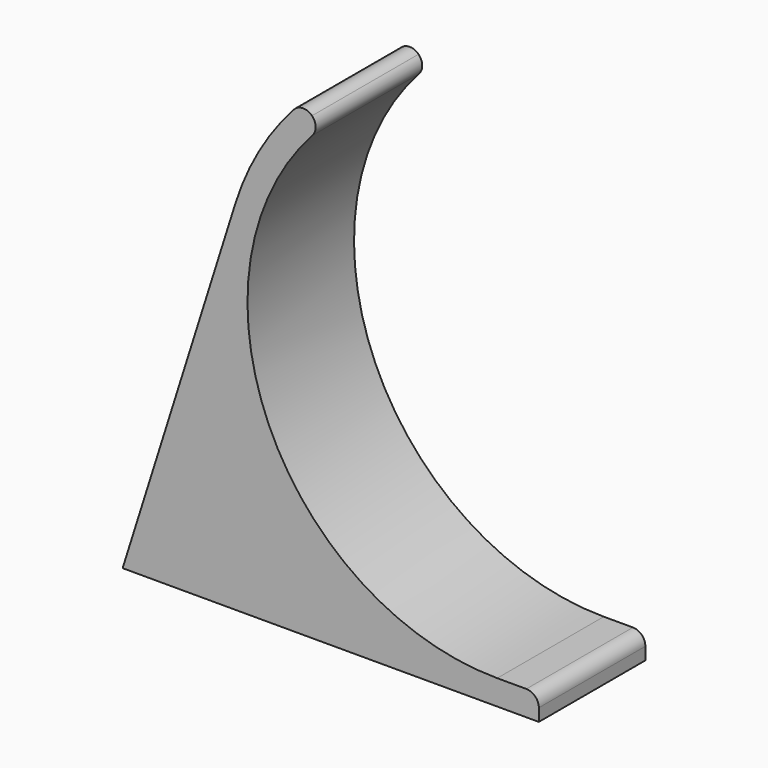
from build123d import *

# Parameters (mm, degrees)
F1_DEPTH = 16
F2_R     = 1.49999


# Not quite as in the source:
# - a fillet or chamfer is up to 0.001 mm smaller than in the source, because OpenCascade refuses the exact size


with BuildPart() as f1:
    # F0 (on Front) → F1 (new body)
    with BuildSketch(Plane.XZ):
        with BuildLine():
            ThreePointArc((0, -33), (-26.6113648632, -19.5150008997), (-31.4739884393, 9.9190751445))
            Line((-31.4739884393, 9.9190751445), (-45, -33))
            Line((-45, -33), (0, -33))
        make_face()
        with BuildLine():
            Line((5, -30), (0, -30))
            ThreePointArc((0, -30), (-27.7163859753, -11.480502971), (-21.2132034356, 21.2132034356))
            Line((-21.2132034356, 21.2132034356), (-23.3345237792, 23.3345237792))
            ThreePointArc((-23.3345237792, 23.3345237792), (-28.213238354, 17.1176278024), (-31.4739884393, 9.9190751445))
            ThreePointArc((-31.4739884393, 9.9190751445), (-26.6113648632, -19.5150008997), (0, -33))
            ThreePointArc((0, -33), (2.5072470561, -32.9046153632), (5, -32.6190128606))
            Line((5, -32.6190128606), (5, -30))
        make_face()
        with BuildLine():
            Line((5, -33), (5, -32.6190128606))
            ThreePointArc((5, -32.6190128606), (2.5072470561, -32.9046153632), (0, -33))
            Line((0, -33), (5, -33))
        make_face()
    extrude(amount=F1_DEPTH)

    # F2 (radius 1.5 in the source; OpenCascade refuses exactly that, so slightly less here)
    f2_edges = [f1.edges().sort_by_distance(p)[0] for p in [
        (-21.213203, -8, 21.213203),
        (-23.334524, -8, 23.334524),
        (5, -8, -30),
    ]]
    fillet(f2_edges, radius=F2_R)


solid = f1.part
